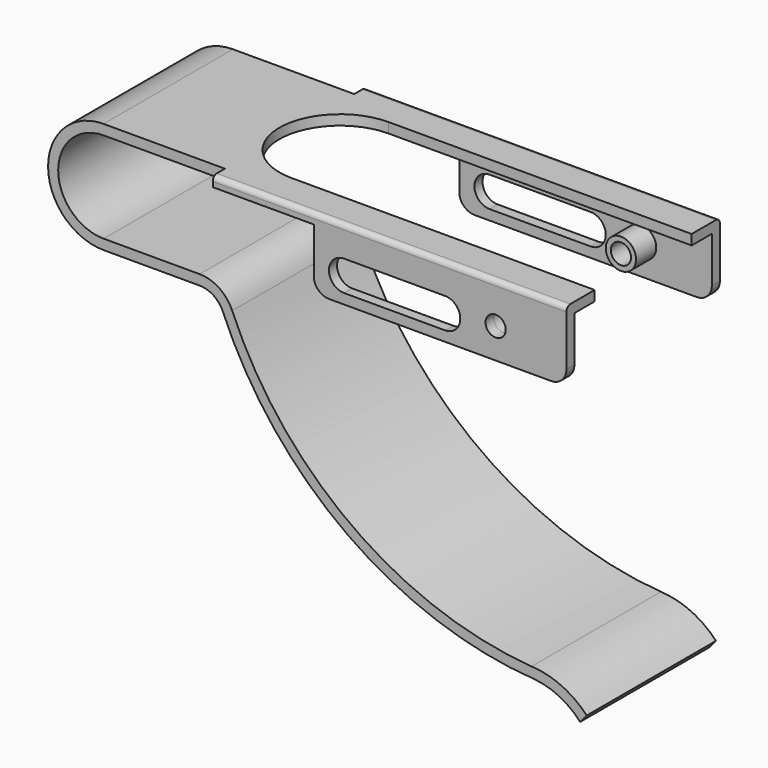
from build123d import *

# Parameters (mm, degrees)
F1_DEPTH  = 16
F2_W      = 70
F2_H      = 3
F3_DEPTH  = 2
F4_W      = 50
F4_H      = 14
F5_DEPTH  = 2
F6_R      = 1
F9_DEPTH  = 2
F11_DEPTH = 38.001
F13_D     = 4
F14_R     = 3
F14_R_2   = 2
F15_DEPTH = 5
F16_R     = 3


# Not quite as in the source:
# - a pattern or mirror of a feature is missing from the dataset's text; its kind, count and spacing are read off the source's solid


with BuildPart() as f1:
    # F0 (on Front) → F1 (new body)
    with BuildSketch(Plane.XZ):
        with BuildLine():
            Line((94, 11), (0, 11))
            ThreePointArc((0, 11), (-11, 0), (0, -11))
            Line((0, -11), (19, -11))
            ThreePointArc((19, -11), (21.7681124643, -11.8361612201), (23.6103896104, -14.064978646))
            ThreePointArc((23.6103896104, -14.064978646), (48.2280702466, -44.8445615778), (85.3629298173, -58.0511936248))
            ThreePointArc((85.3629298173, -58.0511936248), (90.2653686658, -59.4661290396), (94.3351335924, -62.5439468273))
            Line((94.3351335924, -62.5439468273), (95.6306588057, -61))
            ThreePointArc((95.6306588057, -61), (90.6542803924, -57.4351678896), (84.7034264019, -56))
            ThreePointArc((84.7034264019, -56), (49.0672193413, -42.9854179344), (25.4545454545, -13.2909701044))
            ThreePointArc((25.4545454545, -13.2909701044), (22.87535745, -10.1706257081), (19, -9))
            Line((19, -9), (0, -9))
            ThreePointArc((0, -9), (-9, 0), (0, 9))
            Line((0, 9), (94, 9))
            Line((94, 9), (94, 11))
        make_face()
    extrude(amount=F1_DEPTH)

    # F2 (on face) → F3 (join)
    with BuildSketch(Plane.XY.offset(11)):
        with Locations((59, -17.5)):
            Rectangle(F2_W, F2_H)
    extrude(amount=-F3_DEPTH)

    # F4 (on face) → F5 (join)
    with BuildSketch(Plane.XZ.offset(19)):
        with Locations((69, 4)):
            Rectangle(F4_W, F4_H)
    extrude(amount=-F5_DEPTH)

    # F6
    f6_edges = [f1.edges().sort_by_distance(p)[0] for p in [
        (59, -19, 11),
    ]]
    fillet(f6_edges, radius=F6_R)

    # F7: F1 across plane


with BuildPart() as f1_1:
    add(f1.part)
    add(f1.part.mirror(Plane.XZ))

    # F8 (on face) → F9 (cut)
    with BuildSketch(Plane.XY.offset(11)):
        with BuildLine():
            Line((94, 12), (34, 12))
            ThreePointArc((34, 12), (22.0005037904, 0.1099577956), (33.7800936413, -11.9979848805))
            Line((33.7800936413, -11.9979848805), (34.2199063587, -11.9979848805))
            Line((34.2199063587, -11.9979848805), (94, -11.9979848805))
            Line((94, -11.9979848805), (94, 12))
        make_face()
    extrude(amount=-F9_DEPTH, mode=Mode.SUBTRACT)

    # F10 (on face) → F11 (cut, through all)
    with BuildSketch(Plane.XZ.offset(19)):
        with BuildLine():
            ThreePointArc((50, 5), (47, 2), (50, -1))
            Line((50, -1), (70, -1))
            ThreePointArc((70, -1), (73, 2), (70, 5))
            Line((70, 5), (50, 5))
        make_face()
    extrude(amount=-F11_DEPTH, mode=Mode.SUBTRACT)

    # F13 (through all)
    with Locations(Plane.XZ.offset(19)):
        with Locations((80, 3)):
            Hole(F13_D / 2)

    # F14 (on face) → F15 (join)
    with BuildSketch(Plane(origin=(0, -17, 0), x_dir=(-1, 0, 0), z_dir=(0, 1, 0))):
        with Locations((-80, 3)):
            Circle(F14_R)
        with Locations((-80, 3)):
            Circle(F14_R_2, mode=Mode.SUBTRACT)
    f15 = extrude(amount=F15_DEPTH)

    # F15_copies: F15 across plane
    add(f15.mirror(Plane.ZX))

    # F16
    f16_edges = [f1_1.edges().sort_by_distance(p)[0] for p in [
        (94, -18, -3),
        (44, -18, -3),
        (44, 18, -3),
        (94, 18, -3),
    ]]
    fillet(f16_edges, radius=F16_R)


solid = f1_1.part
